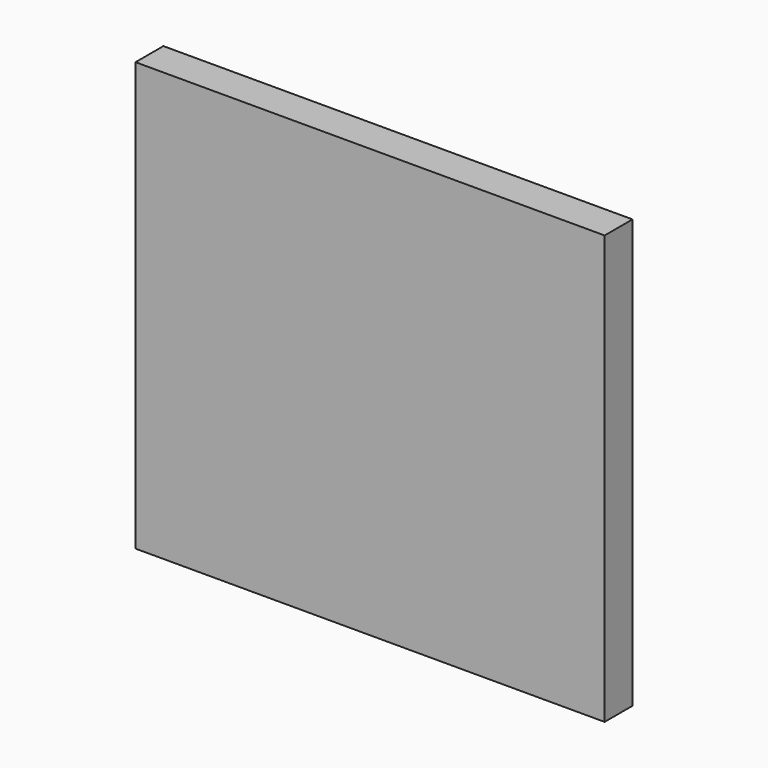
from build123d import *

# Parameters (mm, degrees)
F1_E2_RIGHT_W = 87.4209739268
F1_E2_RIGHT_H = 7.112
F2_DEPTH      = 95.758


with BuildPart() as f2:
    # F1_E2_right (on explicit) → F2 (new body)
    with BuildSketch(Plane(origin=(-55.6937977672, 0, -34.7623750567), x_dir=(0, 0, 1), z_dir=(-1, 0, 0))):
        with Locations((43.7104869634, 3.556)):
            Rectangle(F1_E2_RIGHT_W, F1_E2_RIGHT_H)
    extrude(amount=-F2_DEPTH)


solid = f2.part
